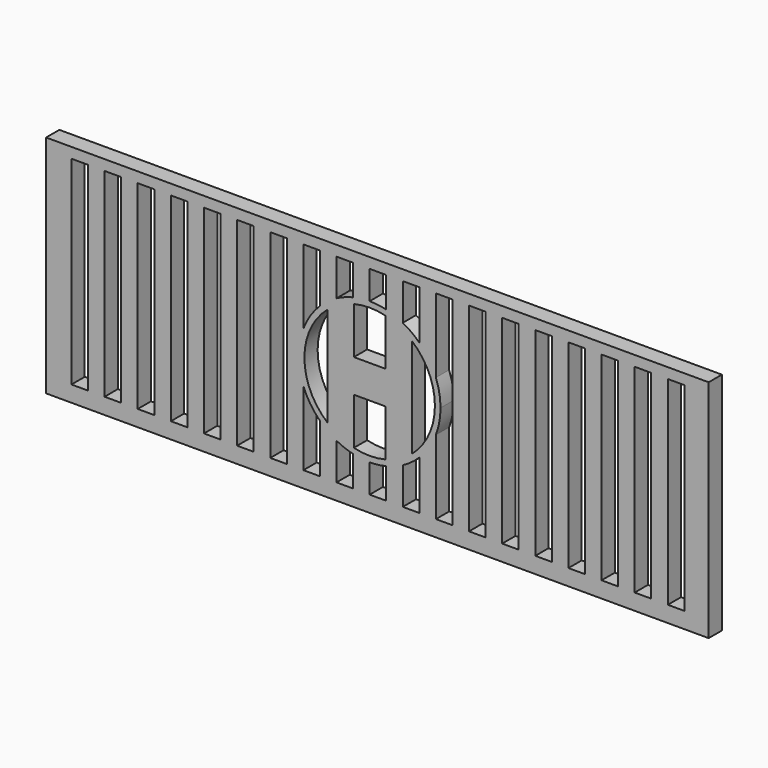
from build123d import *

# Parameters (mm, degrees)
F0_W     = 508
F0_H     = 172.72
F0_W_2   = 12.7
F0_H_2   = 152.4
F1_DEPTH = 12.7


# Not quite as in the source:
# - a feature names something its author has since deleted; it is built from what else it names


with BuildPart() as f1:
    # F0 (on Front) → F1 (new body)
    with BuildSketch(Plane.XZ):
        with Locations((5.9242316484, -2.1814669756)):
            Rectangle(F0_W, F0_H)
        Polygon((215.9, 76.2), (228.6, 76.2), (241.3, 76.2), (241.3, -76.2), (228.6, -76.2), (215.9, -76.2), (203.2, -76.2), (190.5, -76.2), (177.8, -76.2), (165.1, -76.2), (152.4, -76.2), (139.7, -76.2), (127, -76.2), (114.3, -76.2), (101.6, -76.2), (88.9, -76.2), (76.2, -76.2), (63.5, -76.2), (50.8, -76.2), (38.1, -76.2), (25.4, -76.2), (12.7, -76.2), (0, -76.2), (-12.7, -76.2), (-25.4, -76.2), (-38.1, -76.2), (-50.8, -76.2), (-63.5, -76.2), (-76.2, -76.2), (-88.9, -76.2), (-101.6, -76.2), (-114.3, -76.2), (-127, -76.2), (-139.7, -76.2), (-152.4, -76.2), (-165.1, -76.2), (-177.8, -76.2), (-190.5, -76.2), (-203.2, -76.2), (-215.9, -76.2), (-228.6, -76.2), (-228.6, 76.2), (-215.9, 76.2), (-203.2, 76.2), (-190.5, 76.2), (-177.8, 76.2), (-165.1, 76.2), (-152.4, 76.2), (-139.7, 76.2), (-127, 76.2), (-114.3, 76.2), (-101.6, 76.2), (-88.9, 76.2), (-76.2, 76.2), (-63.5, 76.2), (-50.8, 76.2), (-38.1, 76.2), (-25.4, 76.2), (-12.7, 76.2), (0, 76.2), (12.7, 76.2), (25.4, 76.2), (38.1, 76.2), (50.8, 76.2), (63.5, 76.2), (76.2, 76.2), (88.9, 76.2), (101.6, 76.2), (114.3, 76.2), (127, 76.2), (139.7, 76.2), (152.4, 76.2), (165.1, 76.2), (177.8, 76.2), (190.5, 76.2), (203.2, 76.2), align=None, mode=Mode.SUBTRACT)
        with BuildLine():
            ThreePointArc((54.3560246605, 0), (53.4596271482, 9.8308535779), (50.8, 19.3374614904))
            ThreePointArc((50.8, 19.3374614904), (45.4993423984, 29.7386492331), (38.1, 38.7681237216))
            ThreePointArc((38.1, 38.7681237216), (32.0878561317, 43.8742168678), (25.4, 48.056398293))
            ThreePointArc((25.4, 48.056398293), (19.2002837078, 50.8520060807), (12.7, 52.8515602125))
            ThreePointArc((12.7, 52.8515602125), (6.3944001532, 53.9785981994), (0, 54.3560246605))
            ThreePointArc((0, 54.3560246605), (-6.3944001532, 53.9785981994), (-12.7, 52.8515602125))
            ThreePointArc((-12.7, 52.8515602125), (-19.2002837078, 50.8520060807), (-25.4, 48.056398293))
            ThreePointArc((-25.4, 48.056398293), (-32.0878561317, 43.8742168678), (-38.1, 38.7681237216))
            ThreePointArc((-38.1, 38.7681237216), (-45.4993423984, 29.7386492331), (-50.8, 19.3374614904))
            ThreePointArc((-50.8, 19.3374614904), (-54.3560246605, 0), (-50.8, -19.3374614904))
            ThreePointArc((-50.8, -19.3374614904), (-45.4993423984, -29.7386492331), (-38.1, -38.7681237216))
            ThreePointArc((-38.1, -38.7681237216), (-32.0878561317, -43.8742168678), (-25.4, -48.056398293))
            ThreePointArc((-25.4, -48.056398293), (-19.2002837078, -50.8520060807), (-12.7, -52.8515602125))
            ThreePointArc((-12.7, -52.8515602125), (-6.3944001532, -53.9785981994), (0, -54.3560246605))
            ThreePointArc((0, -54.3560246605), (6.3944001532, -53.9785981994), (12.7, -52.8515602125))
            ThreePointArc((12.7, -52.8515602125), (19.2002837078, -50.8520060807), (25.4, -48.056398293))
            ThreePointArc((25.4, -48.056398293), (32.0878561317, -43.8742168678), (38.1, -38.7681237216))
            ThreePointArc((38.1, -38.7681237216), (45.4993423984, -29.7386492331), (50.8, -19.3374614904))
            ThreePointArc((50.8, -19.3374614904), (53.4596271482, -9.8308535779), (54.3560246605, 0))
        make_face()
        with BuildLine():
            ThreePointArc((32.4163123757, 38.1), (45.4094130092, 20.9860076765), (50.0242671914, 0))
            ThreePointArc((50.0242671914, 0), (45.4094130092, -20.9860076765), (32.4163123757, -38.1))
            ThreePointArc((32.4163123757, -38.1), (22.8602382496, -44.4953572321), (12.0963123757, -48.5397418097))
            ThreePointArc((12.0963123757, -48.5397418097), (0, -50.0242671914), (-12.0963123757, -48.5397418097))
            ThreePointArc((-12.0963123757, -48.5397418097), (-22.8602382496, -44.4953572321), (-32.4163123757, -38.1))
            ThreePointArc((-32.4163123757, -38.1), (-50.0242671914, 0), (-32.4163123757, 38.1))
            ThreePointArc((-32.4163123757, 38.1), (-22.8602382496, 44.4953572321), (-12.0963123757, 48.5397418097))
            ThreePointArc((-12.0963123757, 48.5397418097), (0, 50.0242671914), (12.0963123757, 48.5397418097))
            ThreePointArc((12.0963123757, 48.5397418097), (22.8602382496, 44.4953572321), (32.4163123757, 38.1))
        make_face(mode=Mode.SUBTRACT)
        Polygon((32.4163123757, -38.1), (32.4163123757, 38.1), (12.0963123757, 38.1), (12.0963123757, 12.7), (-12.0963123757, 12.7), (-12.0963123757, 38.1), (-32.4163123757, 38.1), (-32.4163123757, -38.1), (-12.0963123757, -38.1), (-12.0963123757, -12.7), (12.0963123757, -12.7), (12.0963123757, -38.1), align=None)
        with Locations((-209.55, 0)):
            Rectangle(F0_W_2, F0_H_2)
        with Locations((-184.15, 0)):
            Rectangle(F0_W_2, F0_H_2)
        with Locations((-158.75, 0)):
            Rectangle(F0_W_2, F0_H_2)
        with Locations((-133.35, 0)):
            Rectangle(F0_W_2, F0_H_2)
        with Locations((-107.95, 0)):
            Rectangle(F0_W_2, F0_H_2)
        with Locations((-82.55, 0)):
            Rectangle(F0_W_2, F0_H_2)
        with Locations((69.85, 0)):
            Rectangle(F0_W_2, F0_H_2)
        with Locations((95.25, 0)):
            Rectangle(F0_W_2, F0_H_2)
        with Locations((120.65, 0)):
            Rectangle(F0_W_2, F0_H_2)
        with Locations((146.05, 0)):
            Rectangle(F0_W_2, F0_H_2)
        with Locations((171.45, 0)):
            Rectangle(F0_W_2, F0_H_2)
        with Locations((196.85, 0)):
            Rectangle(F0_W_2, F0_H_2)
        with Locations((222.25, 0)):
            Rectangle(F0_W_2, F0_H_2)
        with BuildLine():
            Line((-50.8, 19.3374614904), (-50.8, 76.2))
            Line((-50.8, 76.2), (-63.5, 76.2))
            Line((-63.5, 76.2), (-63.5, -76.2))
            Line((-63.5, -76.2), (-50.8, -76.2))
            Line((-50.8, -76.2), (-50.8, -19.3374614904))
            ThreePointArc((-50.8, -19.3374614904), (-54.3560246605, 0), (-50.8, 19.3374614904))
        make_face()
        with BuildLine():
            Line((50.8, 19.3374614904), (50.8, 76.2))
            Line((50.8, 76.2), (38.1, 76.2))
            Line((38.1, 76.2), (38.1, 38.7681237216))
            ThreePointArc((38.1, 38.7681237216), (45.4993423984, 29.7386492331), (50.8, 19.3374614904))
        make_face()
        with BuildLine():
            Line((38.1, -76.2), (50.8, -76.2))
            Line((50.8, -76.2), (50.8, -19.3374614904))
            ThreePointArc((50.8, -19.3374614904), (45.4993423984, -29.7386492331), (38.1, -38.7681237216))
            Line((38.1, -38.7681237216), (38.1, -76.2))
        make_face()
        with BuildLine():
            Line((-25.4, 48.056398293), (-25.4, 76.2))
            Line((-25.4, 76.2), (-38.1, 76.2))
            Line((-38.1, 76.2), (-38.1, 38.7681237216))
            ThreePointArc((-38.1, 38.7681237216), (-32.0878561317, 43.8742168678), (-25.4, 48.056398293))
        make_face()
        with BuildLine():
            Line((-38.1, -76.2), (-25.4, -76.2))
            Line((-25.4, -76.2), (-25.4, -48.056398293))
            ThreePointArc((-25.4, -48.056398293), (-32.0878561317, -43.8742168678), (-38.1, -38.7681237216))
            Line((-38.1, -38.7681237216), (-38.1, -76.2))
        make_face()
        with BuildLine():
            Line((25.4, 48.056398293), (25.4, 76.2))
            Line((25.4, 76.2), (12.7, 76.2))
            Line((12.7, 76.2), (12.7, 52.8515602125))
            ThreePointArc((12.7, 52.8515602125), (19.2002837078, 50.8520060807), (25.4, 48.056398293))
        make_face()
        with BuildLine():
            Line((12.7, -76.2), (25.4, -76.2))
            Line((25.4, -76.2), (25.4, -48.056398293))
            ThreePointArc((25.4, -48.056398293), (19.2002837078, -50.8520060807), (12.7, -52.8515602125))
            Line((12.7, -52.8515602125), (12.7, -76.2))
        make_face()
        with BuildLine():
            Line((0, 54.3560246605), (0, 76.2))
            Line((0, 76.2), (-12.7, 76.2))
            Line((-12.7, 76.2), (-12.7, 52.8515602125))
            ThreePointArc((-12.7, 52.8515602125), (-6.3944001532, 53.9785981994), (0, 54.3560246605))
        make_face()
        with BuildLine():
            Line((-12.7, -76.2), (0, -76.2))
            Line((0, -76.2), (0, -54.3560246605))
            ThreePointArc((0, -54.3560246605), (-6.3944001532, -53.9785981994), (-12.7, -52.8515602125))
            Line((-12.7, -52.8515602125), (-12.7, -76.2))
        make_face()
        with BuildLine():
            Line((-12.0963123757, 38.1), (-12.0963123757, 48.5397418097))
            ThreePointArc((-12.0963123757, 48.5397418097), (-22.8602382496, 44.4953572321), (-32.4163123757, 38.1))
            Line((-32.4163123757, 38.1), (-12.0963123757, 38.1))
        make_face()
        with BuildLine():
            Line((12.0963123757, 38.1), (32.4163123757, 38.1))
            ThreePointArc((32.4163123757, 38.1), (22.8602382496, 44.4953572321), (12.0963123757, 48.5397418097))
            Line((12.0963123757, 48.5397418097), (12.0963123757, 38.1))
        make_face()
        with BuildLine():
            ThreePointArc((12.0963123757, -48.5397418097), (22.8602382496, -44.4953572321), (32.4163123757, -38.1))
            Line((32.4163123757, -38.1), (12.0963123757, -38.1))
            Line((12.0963123757, -38.1), (12.0963123757, -48.5397418097))
        make_face()
        with BuildLine():
            ThreePointArc((-32.4163123757, -38.1), (-22.8602382496, -44.4953572321), (-12.0963123757, -48.5397418097))
            Line((-12.0963123757, -48.5397418097), (-12.0963123757, -38.1))
            Line((-12.0963123757, -38.1), (-32.4163123757, -38.1))
        make_face()
    extrude(amount=F1_DEPTH)


solid = f1.part
